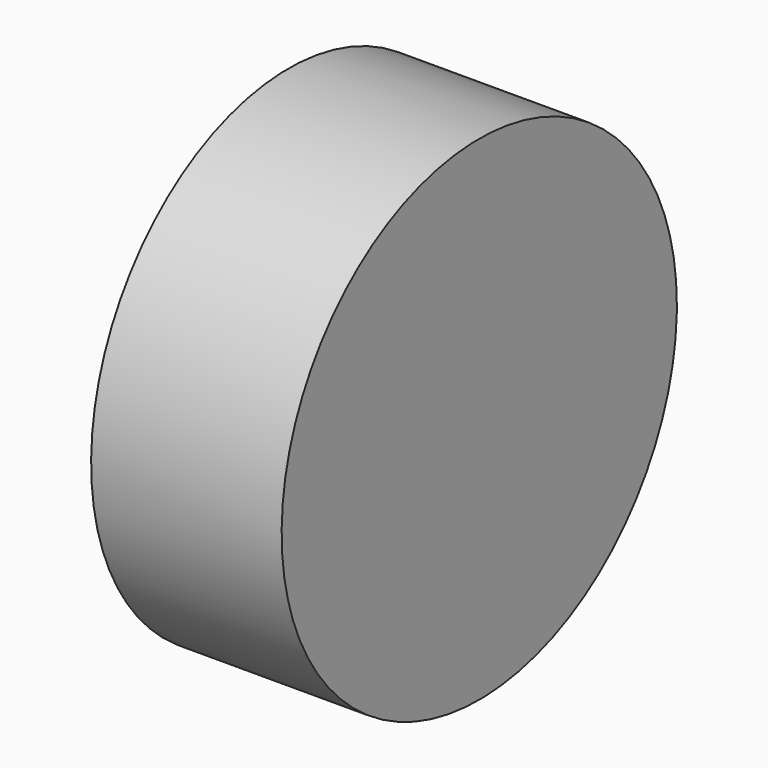
from build123d import *

# Parameters (mm, degrees)
F0_W      = 67.9279565811
F0_H      = 88.0647003651
F1_DEPTH  = 2.54
F1_FACE_W = 67.9279565811
F1_FACE_H = 88.0647003651


# Not quite as in the source:
# - a feature of the source that left no trace in its solid (it failed there, or was rolled back) is left out


with BuildPart() as f1:
    # F0 (on Top) → F1 (new body)
    with BuildSketch(Plane.XY):
        Rectangle(F0_W, F0_H)
    extrude(amount=F1_DEPTH)

    # F1_face (on face) → F2 (revolve)
    with BuildSketch(Plane.XY.offset(2.54)):
        Rectangle(F1_FACE_W, F1_FACE_H)
    revolve(axis=Axis((0, -44.0323501825, 2.54), (-1, 0, 0)))


solid = f1.part
